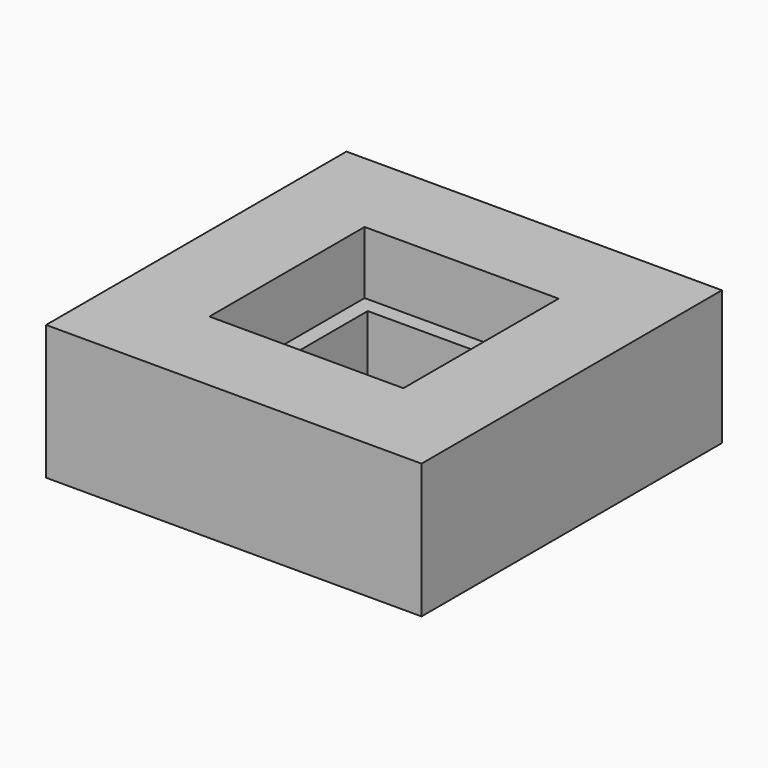
from build123d import *

# Parameters (mm, degrees)
F0_W     = 120
F0_H     = 120
F1_DEPTH = 3
F2_W     = 52
F2_H     = 52
F3_DEPTH = 25
F2_W_2   = 120
F2_H_2   = 120
F2_W_3   = 70
F2_H_3   = 70
F2_R     = 2.5
F4_DEPTH = 37
F5_W     = 120
F5_H     = 120
F5_W_2   = 114
F5_H_2   = 114
F5_W_3   = 52
F5_H_3   = 52
F6_DEPTH = 3
F7_W     = 62
F7_H     = 62
F7_W_2   = 52
F7_H_2   = 52
F8_DEPTH = 20


with BuildPart() as f1:
    # F0 (on Top) → F1 (new body)
    with BuildSketch(Plane.XY):
        Rectangle(F0_W, F0_H)
    extrude(amount=F1_DEPTH)

    # F2 (on face) → F3 (cut)
    with BuildSketch(Plane.XY.offset(3)):
        Rectangle(F2_W, F2_H)
    extrude(amount=-F3_DEPTH, mode=Mode.SUBTRACT)

    # F2 (on face) → F4 (join)
    with BuildSketch(Plane.XY.offset(3)):
        Rectangle(F2_W_2, F2_H_2)
        Polygon((-57, -57), (-57, -35), (-57, 35), (-57, 57), (-35, 57), (35, 57), (57, 57), (57, 35), (57, -35), (57, -57), (35, -57), (-35, -57), align=None, mode=Mode.SUBTRACT)
        Rectangle(F2_W_3, F2_H_3)
        Rectangle(F2_W, F2_H, mode=Mode.SUBTRACT)
        with Locations((46, 46)):
            Circle(F2_R)
        with Locations((0, 46)):
            Circle(F2_R)
        with Locations((-46, 46)):
            Circle(F2_R)
        with Locations((-46, 0)):
            Circle(F2_R)
        with Locations((-46, -46)):
            Circle(F2_R)
        with Locations((0, -46)):
            Circle(F2_R)
        with Locations((46, -46)):
            Circle(F2_R)
        with Locations((46, 0)):
            Circle(F2_R)
    extrude(amount=F4_DEPTH)

    # F5 (on face) → F6 (join)
    with BuildSketch(Plane.XY.offset(40)):
        Rectangle(F5_W, F5_H)
        Rectangle(F5_W_2, F5_H_2, mode=Mode.SUBTRACT)
        Rectangle(F5_W_2, F5_H_2)
        Rectangle(F5_W_3, F5_H_3, mode=Mode.SUBTRACT)
    extrude(amount=F6_DEPTH)

    # F7 (on face) → F8 (cut)
    with BuildSketch(Plane.XY.offset(43)):
        Rectangle(F7_W, F7_H)
        Rectangle(F7_W_2, F7_H_2, mode=Mode.SUBTRACT)
    extrude(amount=-F8_DEPTH, mode=Mode.SUBTRACT)


solid = f1.part
